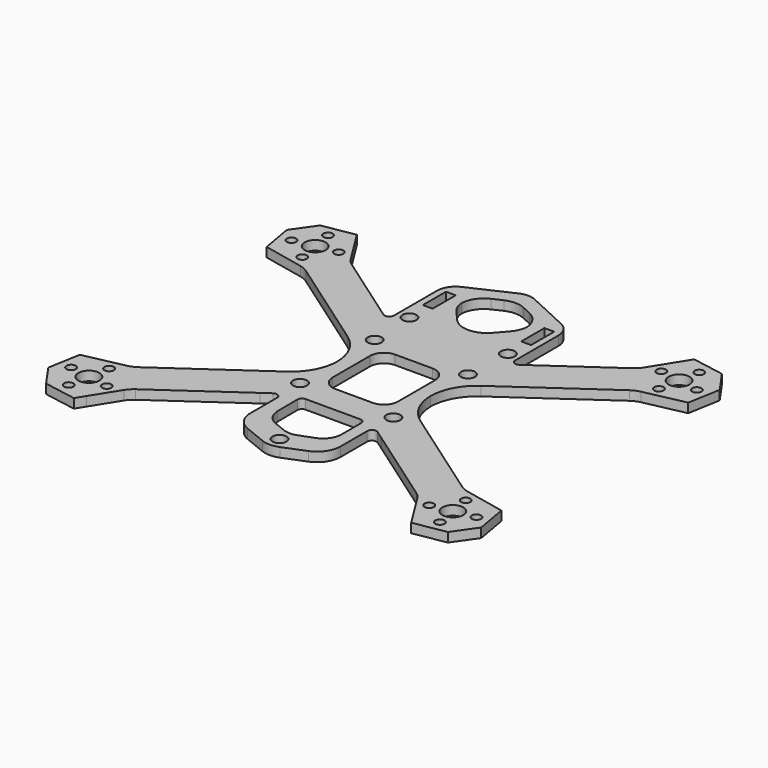
from build123d import *

# Parameters (mm, degrees)
F0_R         = 1.5
F0_R_2       = 1
F0_R_3       = 2.25
F0_W         = 2.1
F0_H         = 6.2
F1_DEPTH     = 2
F3_DEPTH     = 2
F4_R         = 4
F6_DEPTH     = 2.001
F7_T1_DEPTH  = 2
F9_DEPTH     = 2.001
F10_R        = 5
F11_R        = 1
F12_T1_DEPTH = 2
F14_DEPTH    = 2
F16_DEPTH    = 2.001
F18_DEPTH    = 2.001
F19_R        = 5
F21_DEPTH    = 2.001
F22_R        = 4
F23_R        = 1
F24_R        = 1


# Not quite as in the source:
# - a fillet or chamfer that OpenCascade refuses, or shapes differently, is made with other operations: its cross-section is extruded or revolved along the edge and cut away or added


with BuildPart() as f1:
    # F0 (on Top) → F1 (new body)
    with BuildSketch(Plane.XY):
        Polygon((13, 3.5572758754), (13, 13), (-13, 13), (-13, 3.5572758754), (-13, -3.5572758754), (-13, -13), (13, -13), (13, -3.5572758754), align=None)
        with Locations((-10, -10)):
            Circle(F0_R, mode=Mode.SUBTRACT)
        with Locations((10, -10)):
            Circle(F0_R, mode=Mode.SUBTRACT)
        with Locations((-10, 10)):
            Circle(F0_R, mode=Mode.SUBTRACT)
        with Locations((10, 10)):
            Circle(F0_R, mode=Mode.SUBTRACT)
        with BuildLine():
            Line((13, 20.6481201181), (13, 13))
            Line((13, 13), (13, 3.5572758754))
            Line((13, 3.5572758754), (43.0150350545, 24.5740296802))
            ThreePointArc((43.0150350545, 24.5740296802), (44.73406431, 34.3231290446), (34.9849649455, 36.0421583002))
            Line((34.9849649455, 36.0421583002), (13, 20.6481201181))
        make_face()
        with Locations((38.2185832005, 25.8764591016)):
            Circle(F0_R_2, mode=Mode.SUBTRACT)
        with Locations((39, 30.3080939902)):
            Circle(F0_R_3, mode=Mode.SUBTRACT)
        with Locations((34.5683651114, 31.0895107897)):
            Circle(F0_R_2, mode=Mode.SUBTRACT)
        with Locations((43.4316348886, 29.5266771907)):
            Circle(F0_R_2, mode=Mode.SUBTRACT)
        with Locations((39.7814167995, 34.7397288787)):
            Circle(F0_R_2, mode=Mode.SUBTRACT)
        Polygon((-13, 13), (13, 13), (13, 20.6481201181), (13, 33), (-13, 33), (-13, 20.6481201181), align=None)
        with Locations((-10.55, 20)):
            Circle(F0_R, mode=Mode.SUBTRACT)
        with Locations((-10.55, 28)):
            Rectangle(F0_W, F0_H, mode=Mode.SUBTRACT)
        with Locations((10.55, 20)):
            Circle(F0_R, mode=Mode.SUBTRACT)
        with Locations((10.55, 28)):
            Rectangle(F0_W, F0_H, mode=Mode.SUBTRACT)
        with BuildLine():
            Line((-13, 3.5572758754), (-13, 13))
            Line((-13, 13), (-13, 20.6481201181))
            Line((-13, 20.6481201181), (-34.9849649455, 36.0421583002))
            ThreePointArc((-34.9849649455, 36.0421583002), (-44.73406431, 34.3231290446), (-43.0150350545, 24.5740296802))
            Line((-43.0150350545, 24.5740296802), (-13, 3.5572758754))
        make_face()
        with Locations((-38.2185832005, 25.8764591016)):
            Circle(F0_R_2, mode=Mode.SUBTRACT)
        with Locations((-43.4316348886, 29.5266771907)):
            Circle(F0_R_2, mode=Mode.SUBTRACT)
        with Locations((-39, 30.3080939902)):
            Circle(F0_R_3, mode=Mode.SUBTRACT)
        with Locations((-34.5683651114, 31.0895107897)):
            Circle(F0_R_2, mode=Mode.SUBTRACT)
        with Locations((-39.7814167995, 34.7397288787)):
            Circle(F0_R_2, mode=Mode.SUBTRACT)
        with BuildLine():
            Line((43.0150350545, -24.5740296802), (13, -3.5572758754))
            Line((13, -3.5572758754), (13, -13))
            Line((13, -13), (13, -20.6481201181))
            Line((13, -20.6481201181), (34.9849649455, -36.0421583002))
            ThreePointArc((34.9849649455, -36.0421583002), (44.73406431, -34.3231290446), (43.0150350545, -24.5740296802))
        make_face()
        with Locations((39.7814167995, -34.7397288787)):
            Circle(F0_R_2, mode=Mode.SUBTRACT)
        with Locations((34.5683651114, -31.0895107897)):
            Circle(F0_R_2, mode=Mode.SUBTRACT)
        with Locations((39, -30.3080939902)):
            Circle(F0_R_3, mode=Mode.SUBTRACT)
        with Locations((43.4316348886, -29.5266771907)):
            Circle(F0_R_2, mode=Mode.SUBTRACT)
        with Locations((38.2185832005, -25.8764591016)):
            Circle(F0_R_2, mode=Mode.SUBTRACT)
        with BuildLine():
            Line((-13, -13), (-13, -3.5572758754))
            Line((-13, -3.5572758754), (-43.0150350545, -24.5740296802))
            ThreePointArc((-43.0150350545, -24.5740296802), (-44.73406431, -34.3231290446), (-34.9849649455, -36.0421583002))
            Line((-34.9849649455, -36.0421583002), (-13, -20.6481201181))
            Line((-13, -20.6481201181), (-13, -13))
        make_face()
        with Locations((-39.7814167995, -34.7397288787)):
            Circle(F0_R_2, mode=Mode.SUBTRACT)
        with Locations((-43.4316348886, -29.5266771907)):
            Circle(F0_R_2, mode=Mode.SUBTRACT)
        with Locations((-34.5683651114, -31.0895107897)):
            Circle(F0_R_2, mode=Mode.SUBTRACT)
        with Locations((-39, -30.3080939902)):
            Circle(F0_R_3, mode=Mode.SUBTRACT)
        with Locations((-38.2185832005, -25.8764591016)):
            Circle(F0_R_2, mode=Mode.SUBTRACT)
        Polygon((13, -20.6481201181), (13, -13), (-13, -13), (-13, -20.6481201181), (-13, -31), (13, -31), align=None)
        with Locations((0, -28)):
            Circle(F0_R, mode=Mode.SUBTRACT)
    extrude(amount=F1_DEPTH)

    # F2 (on face) → F3 (join, through all)
    with BuildSketch(Plane.XY.offset(2)):
        Polygon((0, 39), (-13, 33), (-13, 32), (13, 32), (13, 33), align=None)
    extrude(amount=-F3_DEPTH)

    # F4
    f4_edges = [f1.edges().sort_by_distance(p)[0] for p in [
        (-13, 33, 1),
        (0, 39, 1),
        (13, 33, 1),
    ]]
    fillet(f4_edges, radius=F4_R)

    # F5 (on face) → F6 (cut, through all)
    with BuildSketch(Plane.XY.offset(2)):
        Polygon((7, 32.4651182162), (0, 35.6958874469), (-7, 32.4651182162), (-7, 28), (0, 20), (7, 28), align=None)
    extrude(amount=-F6_DEPTH, mode=Mode.SUBTRACT)

    # F7: fillet of radius 5 on 6 edges, made by hand

    # F7_s2 → F7_t1 (join)
    with BuildSketch(Plane.XY):
        with BuildLine():
            ThreePointArc((2.0952908873, 34.7288301143), (0, 35.1890331918), (-2.0952908873, 34.7288301143))
            Line((-2.0952908873, 34.7288301143), (0, 35.6958874469))
            Line((0, 35.6958874469), (2.0952908873, 34.7288301143))
        make_face()
        with BuildLine():
            ThreePointArc((-4.0952908873, 33.8057531913), (-6.2116774827, 31.9607239362), (-7, 29.2659562688))
            Line((-7, 29.2659562688), (-7, 32.4651182162))
            Line((-7, 32.4651182162), (-4.0952908873, 33.8057531913))
        make_face()
        with BuildLine():
            ThreePointArc((4.0952908873, 33.8057531913), (6.2116774827, 31.9607239362), (7, 29.2659562688))
            Line((7, 29.2659562688), (7, 32.4651182162))
            Line((7, 32.4651182162), (4.0952908873, 33.8057531913))
        make_face()
        with BuildLine():
            ThreePointArc((5.7628834735, 26.5861525412), (6.6805137201, 28.1200422145), (7, 29.8786755805))
            Line((7, 29.8786755805), (7, 28))
            Line((7, 28), (5.7628834735, 26.5861525412))
        make_face()
        with BuildLine():
            ThreePointArc((-7, 29.8786755805), (-6.6805137201, 28.1200422145), (-5.7628834735, 26.5861525412))
            Line((-5.7628834735, 26.5861525412), (-7, 28))
            Line((-7, 28), (-7, 29.8786755805))
        make_face()
        with BuildLine():
            ThreePointArc((-3.7628834735, 24.3004382555), (0, 22.5929612948), (3.7628834735, 24.3004382555))
            Line((3.7628834735, 24.3004382555), (0, 20))
            Line((0, 20), (-3.7628834735, 24.3004382555))
        make_face()
    extrude(amount=F7_T1_DEPTH)

    # F8 (on face) → F9 (cut, through all)
    with BuildSketch(Plane.XY.offset(2)):
        Polygon((-34.9849649455, 36.0421583002), (-30.9162904101, 29.5309179537), (-13, 16.9857963518), (-13, 25.5443952801), (-34.9849649455, 40.9384334622), align=None)
        Polygon((-10, -5.1189770271), (-10, 5.1189770271), (-35.5049019009, 22.9777015993), (-43.0150350545, 24.5740296802), (-43.0150350545, 21.0167538048), (-13, 0), (-43.0150350545, -21.0167538048), (-43.0150350545, -24.5740296802), (-35.5049019009, -22.9777015993), align=None)
        Polygon((13, 25.5443952801), (13, 16.9857963518), (30.9162904101, 29.5309179537), (34.9849649455, 36.0421583002), (34.9849649455, 40.9384334622), align=None)
        Polygon((35.5049019009, 22.9777015993), (10, 5.1189770271), (10, -5.1189770271), (35.5049019009, -22.9777015993), (43.0150350545, -24.5740296802), (43.0150350545, -21.0167538048), (13, 0), (43.0150350545, 21.0167538048), (43.0150350545, 24.5740296802), align=None)
        Polygon((13, -16.9857963518), (13, -25.824060059), (34.9849649455, -41.2180982412), (34.9849649455, -36.0421583002), (30.9162904101, -29.5309179537), align=None)
        Polygon((-13, -16.9857963518), (-30.9162904101, -29.5309179537), (-34.9849649455, -36.0421583002), (-34.9849649455, -41.2180982412), (-13, -25.824060059), align=None)
    extrude(amount=-F9_DEPTH, mode=Mode.SUBTRACT)

    # F10
    f10_edges = [f1.edges().sort_by_distance(p)[0] for p in [
        (30.91629, -29.530918, 1),
        (30.91629, 29.530918, 1),
        (-30.91629, 29.530918, 1),
        (-35.504902, 22.977702, 1),
        (35.504902, 22.977702, 1),
        (-35.504902, -22.977702, 1),
        (-30.91629, -29.530918, 1),
        (35.504902, -22.977702, 1),
    ]]
    fillet(f10_edges, radius=F10_R)

    # F11
    f11_edges = [f1.edges().sort_by_distance(p)[0] for p in [
        (-13, 16.985796, 1),
        (13, 16.985796, 1),
    ]]
    fillet(f11_edges, radius=F11_R)

    # F12: fillet of radius 10 on 4 edges, made by hand

    # F12_s2 → F12_t1 (join)
    with BuildSketch(Plane.XY):
        with BuildLine():
            ThreePointArc((-14.2642356365, 8.1048269644), (-11.1298916682, 4.5307926539), (-10, -0.0866934785))
            Line((-10, -0.0866934785), (-10, 5.1189770271))
            Line((-10, 5.1189770271), (-14.2642356365, 8.1048269644))
        make_face()
        with BuildLine():
            ThreePointArc((-10, 0.0866934785), (-11.1298916682, -4.5307926539), (-14.2642356365, -8.1048269644))
            Line((-14.2642356365, -8.1048269644), (-10, -5.1189770271))
            Line((-10, -5.1189770271), (-10, 0.0866934785))
        make_face()
        with BuildLine():
            ThreePointArc((14.2642356365, 8.1048269644), (11.1298916682, 4.5307926539), (10, -0.0866934785))
            Line((10, -0.0866934785), (10, 5.1189770271))
            Line((10, 5.1189770271), (14.2642356365, 8.1048269644))
        make_face()
        with BuildLine():
            ThreePointArc((10, 0.0866934785), (11.1298916682, -4.5307926539), (14.2642356365, -8.1048269644))
            Line((14.2642356365, -8.1048269644), (10, -5.1189770271))
            Line((10, -5.1189770271), (10, 0.0866934785))
        make_face()
    extrude(amount=F12_T1_DEPTH)

    # F13 (on face) → F14 (join, through all)
    with BuildSketch(Plane.XY.offset(2)):
        with BuildLine():
            Line((-45.1779821171, 25.0337782709), (-41.6937086247, 24.2931730774))
            ThreePointArc((-41.6937086247, 24.2931730774), (-44.3986619113, 34.0882777567), (-34.2691258135, 34.89657622))
            Line((-34.2691258135, 34.89657622), (-36.156758768, 37.9174204152))
            Line((-36.156758768, 37.9174204152), (-43.0709823371, 36.6982562494))
            Line((-43.0709823371, 36.6982562494), (-46.397146283, 31.9480018399))
            Line((-46.397146283, 31.9480018399), (-45.1779821171, 25.0337782709))
        make_face()
        with BuildLine():
            Line((36.156758768, 37.9174204152), (34.2691258135, 34.89657622))
            ThreePointArc((34.2691258135, 34.89657622), (44.3986619113, 34.0882777567), (41.6937086247, 24.2931730774))
            Line((41.6937086247, 24.2931730774), (45.1779821171, 25.0337782709))
            Line((45.1779821171, 25.0337782709), (46.397146283, 31.9480018399))
            Line((46.397146283, 31.9480018399), (43.0709823371, 36.6982562494))
            Line((43.0709823371, 36.6982562494), (36.156758768, 37.9174204152))
        make_face()
        with BuildLine():
            Line((-36.156758768, -37.9174204152), (-34.2691258135, -34.89657622))
            ThreePointArc((-34.2691258135, -34.89657622), (-44.3986619113, -34.0882777567), (-41.6937086247, -24.2931730774))
            Line((-41.6937086247, -24.2931730774), (-45.1779821171, -25.0337782709))
            Line((-45.1779821171, -25.0337782709), (-46.397146283, -31.9480018399))
            Line((-46.397146283, -31.9480018399), (-43.0709823371, -36.6982562494))
            Line((-43.0709823371, -36.6982562494), (-36.156758768, -37.9174204152))
        make_face()
        with BuildLine():
            ThreePointArc((41.6937086247, -24.2931730774), (44.3986619113, -34.0882777567), (34.2691258135, -34.89657622))
            Line((34.2691258135, -34.89657622), (36.156758768, -37.9174204152))
            Line((36.156758768, -37.9174204152), (43.0709823371, -36.6982562494))
            Line((43.0709823371, -36.6982562494), (46.397146283, -31.9480018399))
            Line((46.397146283, -31.9480018399), (45.1779821171, -25.0337782709))
            Line((45.1779821171, -25.0337782709), (41.6937086247, -24.2931730774))
        make_face()
    extrude(amount=-F14_DEPTH)

    # F15 (on face) → F16 (cut, through all)
    with BuildSketch(Plane.XY.offset(2)):
        with BuildLine():
            ThreePointArc((7, 5), (6.1213203436, 7.1213203436), (4, 8))
            Line((4, 8), (-4, 8))
            ThreePointArc((-4, 8), (-6.1213203436, 7.1213203436), (-7, 5))
            Line((-7, 5), (-7, -5))
            ThreePointArc((-7, -5), (-6.1213203436, -7.1213203436), (-4, -8))
            Line((-4, -8), (4, -8))
            ThreePointArc((4, -8), (6.1213203436, -7.1213203436), (7, -5))
            Line((7, -5), (7, 5))
        make_face()
    extrude(amount=-F16_DEPTH, mode=Mode.SUBTRACT)

    # F17 (on face) → F18 (cut, through all)
    with BuildSketch(Plane.XY.offset(2)):
        Polygon((14.5735764364, -34.0217222472), (14.5735764364, -18.0876264345), (9.6586641706, -14.6461678163), (9.6586641706, -27.0976463685), (0, -31), (-9.6586641706, -27.0976463685), (-9.6586641706, -14.6461678163), (-14.5735764364, -18.0876264345), (-14.5735764364, -34.0217222472), align=None)
    extrude(amount=-F18_DEPTH, mode=Mode.SUBTRACT)

    # F19
    f19_edges = [f1.edges().sort_by_distance(p)[0] for p in [
        (0, -31, 1),
        (-9.658664, -27.097646, 1),
        (9.658664, -27.097646, 1),
    ]]
    fillet(f19_edges, radius=F19_R)

    # F20 (on face) → F21 (cut, through all)
    with BuildSketch(Plane.XY.offset(2)):
        Polygon((7.0668010645, -13.9628378529), (-6.6244119044, -13.9628378529), (-6.5461801306, -22.9624978348), (0, -25.6073262866), (7.0668010645, -22.9624978348), align=None)
    extrude(amount=-F21_DEPTH, mode=Mode.SUBTRACT)

    # F22
    f22_edges = [f1.edges().sort_by_distance(p)[0] for p in [
        (-6.54618, -22.962498, 1),
        (0, -25.607326, 1),
        (7.066801, -22.962498, 1),
    ]]
    fillet(f22_edges, radius=F22_R)

    # F23
    f23_edges = [f1.edges().sort_by_distance(p)[0] for p in [
        (-6.624412, -13.962838, 1),
        (7.066801, -13.962838, 1),
    ]]
    fillet(f23_edges, radius=F23_R)

    # F24
    f24_edges = [f1.edges().sort_by_distance(p)[0] for p in [
        (-9.658664, -14.646168, 1),
        (9.658664, -14.646168, 1),
    ]]
    fillet(f24_edges, radius=F24_R)


solid = f1.part
